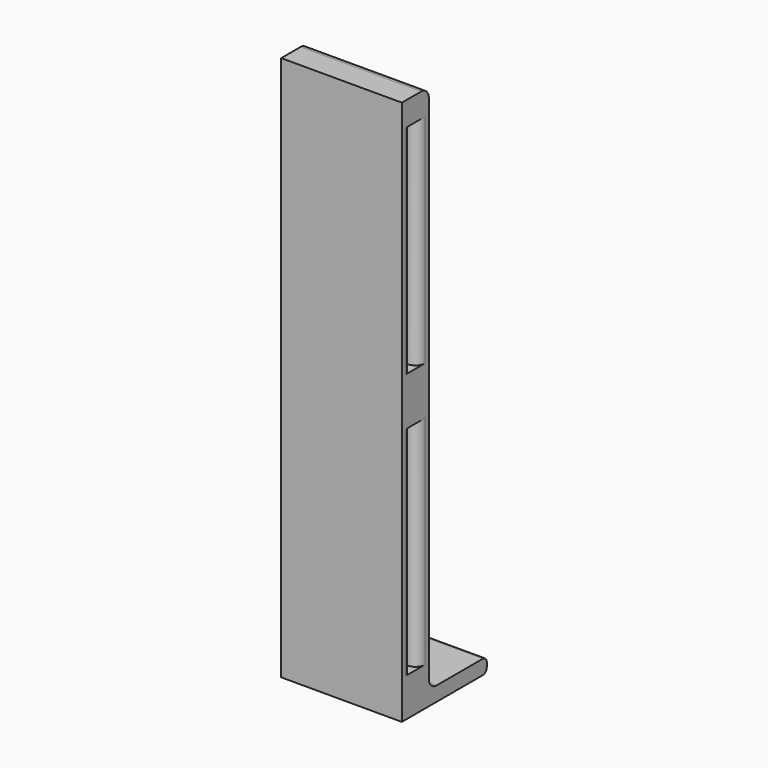
from build123d import *

# Parameters (mm, degrees)
F0_W     = 2
F0_H     = 45
F1_DEPTH = 25
F2_R     = 2
F4_R     = 1


# Not quite as in the source:
# - two fillets or chamfers of one size are made in one step


with BuildPart() as f1:
    # F0 (on Right) → F1 (new body)
    with BuildSketch(Plane.YZ):
        with BuildLine():
            Line((7, 113), (0, 113))
            Line((0, 113), (0, 0))
            Line((0, 0), (21, 0))
            ThreePointArc((21, 0), (21.7071067812, 0.2928932188), (22, 1))
            Line((22, 1), (22, 2))
            ThreePointArc((22, 2), (21.7071067812, 2.7071067812), (21, 3))
            Line((21, 3), (7, 3))
            Line((7, 3), (7, 113))
        make_face()
        with Locations((3, 30.5)):
            Rectangle(F0_W, F0_H, mode=Mode.SUBTRACT)
        with Locations((3, 85.5)):
            Rectangle(F0_W, F0_H, mode=Mode.SUBTRACT)
    extrude(amount=F1_DEPTH)

    # F2 (call 1 of 6: OpenCascade refuses the feature's edges together)
    f2_edges = [f1.edges().sort_by_distance(p)[0] for p in [
        (12.5, 7, 3),
    ]]
    fillet(f2_edges, radius=F2_R)

    # F2#2 (call 2 of 6)
    f2_2_edges = [f1.edges().sort_by_distance(p)[0] for p in [
        (12.5, 7, 113),
    ]]
    fillet(f2_2_edges, radius=F2_R)

    # F2#3 (call 3 of 6)
    f2_3_edges = [f1.edges().sort_by_distance(p)[0] for p in [
        (0, 4, 30.5),
    ]]
    fillet(f2_3_edges, radius=F2_R)

    # F2#4 (call 4 of 6)
    f2_4_edges = [f1.edges().sort_by_distance(p)[0] for p in [
        (25, 4, 30.5),
    ]]
    fillet(f2_4_edges, radius=F2_R)

    # F2#5 (call 5 of 6)
    f2_5_edges = [f1.edges().sort_by_distance(p)[0] for p in [
        (0, 4, 85.5),
    ]]
    fillet(f2_5_edges, radius=F2_R)

    # F2#6 (call 6 of 6)
    f2_6_edges = [f1.edges().sort_by_distance(p)[0] for p in [
        (25, 4, 85.5),
    ]]
    fillet(f2_6_edges, radius=F2_R)

    # F4
    f4_edges = [f1.edges().sort_by_distance(p)[0] for p in [
        (25, 2, 30.5),
        (25, 2, 85.5),
        (0, 2, 85.5),
        (0, 2, 30.5),
    ]]
    fillet(f4_edges, radius=F4_R)


solid = f1.part
